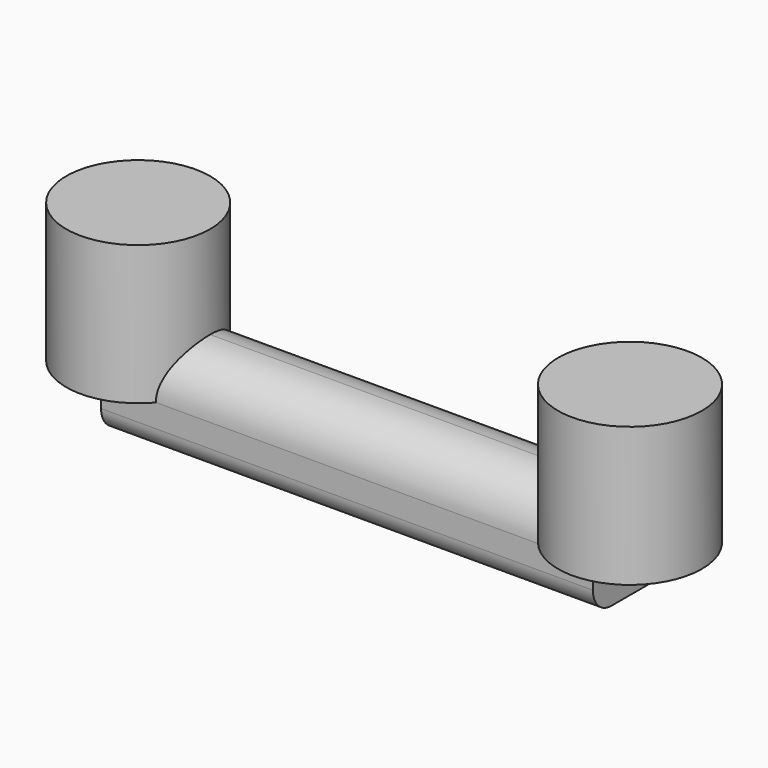
from build123d import *

# Parameters (mm, degrees)
F0_R     = 31
F1_DEPTH = 60
F2_W     = 212
F2_H     = 40
F3_DEPTH = 20
F4_R     = 10
F5_R     = 19.99999


# Not quite as in the source:
# - a fillet or chamfer is up to 0.001 mm smaller than in the source, because OpenCascade refuses the exact size


with BuildPart() as f1:
    # F0 (on Top) → F1 (new body)
    with BuildSketch(Plane.XY):
        with Locations((-106, 0)):
            Circle(F0_R)
    extrude(amount=F1_DEPTH)


with BuildPart() as f1b:
    # F0 (on Top) → F1, piece 2 (new body)
    with BuildSketch(Plane.XY):
        with Locations((106, 0)):
            Circle(F0_R)
    extrude(amount=F1_DEPTH)


with BuildPart() as f3:
    # F2 (on Top) → F3 (new body, symmetric)
    with BuildSketch(Plane.XY):
        Rectangle(F2_W, F2_H)
    extrude(amount=F3_DEPTH, both=True)

    # F4
    f4_edges = [f3.edges().sort_by_distance(p)[0] for p in [
        (0, 20, -20),
        (0, -20, -20),
    ]]
    fillet(f4_edges, radius=F4_R)

    # F5 (radius 20 in the source; OpenCascade refuses exactly that, so slightly less here)
    f5_edges = [f3.edges().sort_by_distance(p)[0] for p in [
        (0, 20, 20),
        (0, -20, 20),
    ]]
    fillet(f5_edges, radius=F5_R)


solid = Compound([f1.part, f1b.part, f3.part])
